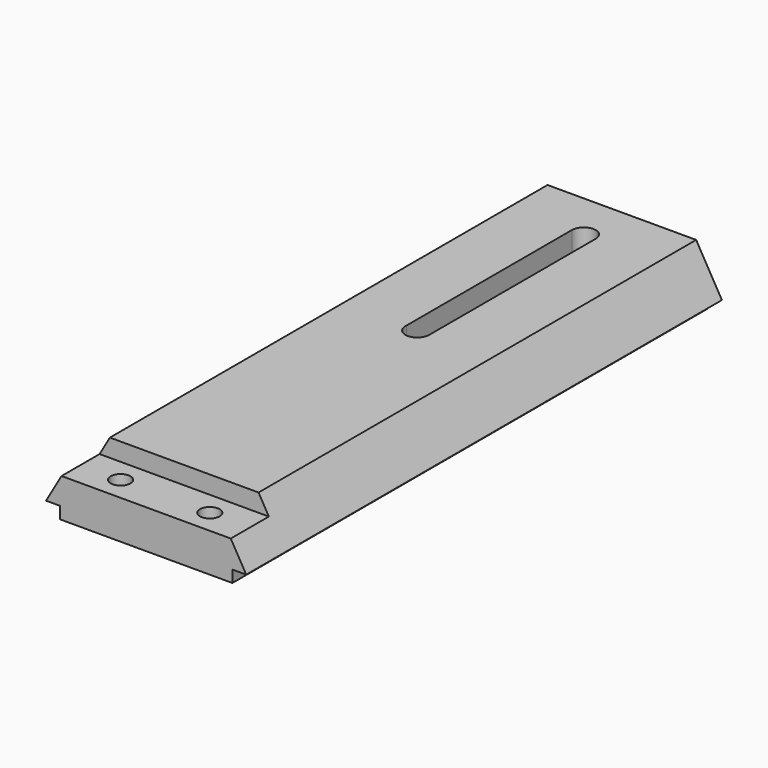
from build123d import *

# Parameters (mm, degrees)
F1_DEPTH   = 50
F1_FACE1_W = 25
F1_FACE1_H = 100
F3_DEPTH   = 6
F5_DEPTH   = 25
F6_W       = 25
F6_H       = 8
F7_DEPTH   = 3
F9_D       = 3.3


with BuildPart() as f1:
    # F0 (on Front) → F1 (new body, symmetric)
    with BuildSketch(Plane.XZ):
        Polygon((-16.8301270189, 2), (-14.5, 2), (-14.5, 0), (14.5, 0), (14.5, 2), (16.8301270189, 2), (12.5, 9.5), (-12.5, 9.5), align=None)
    extrude(amount=F1_DEPTH, both=True)

    # F2 (on face) + F1_face1 (on face) → F3 (cut)
    with BuildSketch(Plane(origin=(0, 0, 0), x_dir=(1, 0, 0), z_dir=(0, 0, -1))):
        with BuildLine():
            Line((4.5, -42), (4.5, -7))
            ThreePointArc((4.5, -7), (0, -2.5), (-4.5, -7))
            Line((-4.5, -7), (-4.5, -42))
            Line((-4.5, -42), (-4.5, -42.0004010455))
            ThreePointArc((-4.4999999821, -42.0004010455), (0.0002005227, -46.4999999955), (4.5, -42))
        make_face()
    with BuildSketch(Plane.XY.offset(9.5)):
        Rectangle(F1_FACE1_W, F1_FACE1_H)
    extrude(amount=-F3_DEPTH, dir=(0, 0, -1), mode=Mode.SUBTRACT)

    # F4 (on face) → F5 (cut)
    with BuildSketch(Plane.XY.offset(9.5)):
        with BuildLine():
            ThreePointArc((-1.9907275363, 7.1923639157), (-0.0962936325, 5.0023194609), (2, 7))
            ThreePointArc((2, 7), (0.0962936325, 8.9976805391), (-1.9907275363, 7.1923639157))
        make_face()
        with BuildLine():
            Line((2, 7), (2, 42))
            ThreePointArc((2, 42), (0.0002663937, 40.0000000177), (-1.999999929, 41.9994672126))
            Line((-1.999999929, 41.9994672126), (-1.9907275363, 7.1923639157))
            ThreePointArc((-1.9907275363, 7.1923639157), (0.0962936325, 8.9976805391), (2, 7))
        make_face()
        with BuildLine():
            ThreePointArc((-1.999999929, 41.9994672126), (0.0002663937, 40.0000000177), (2, 42))
            ThreePointArc((2, 42), (-0.0002663937, 43.9999999823), (-1.999999929, 41.9994672126))
        make_face()
    extrude(amount=-F5_DEPTH, mode=Mode.SUBTRACT)

    # F6 (on face) → F7 (cut)
    with BuildSketch(Plane.XY.offset(9.5)):
        with Locations((0, -46)):
            Rectangle(F6_W, F6_H)
        Polygon((-23.7841614955, -55.5199324694), (24.0457867705, -55.5199324694), (24.0457867705, -42), (12.5, -42), (12.5, -50), (-12.5, -50), (-12.5, -42), (-23.7841614955, -42), align=None)
    extrude(amount=-F7_DEPTH, mode=Mode.SUBTRACT)

    # F9 (through all)
    with Locations(Plane.XY.offset(6.5)):
        with Locations((-7.5, -46), (7.5, -46)):
            Hole(F9_D / 2)


solid = f1.part
